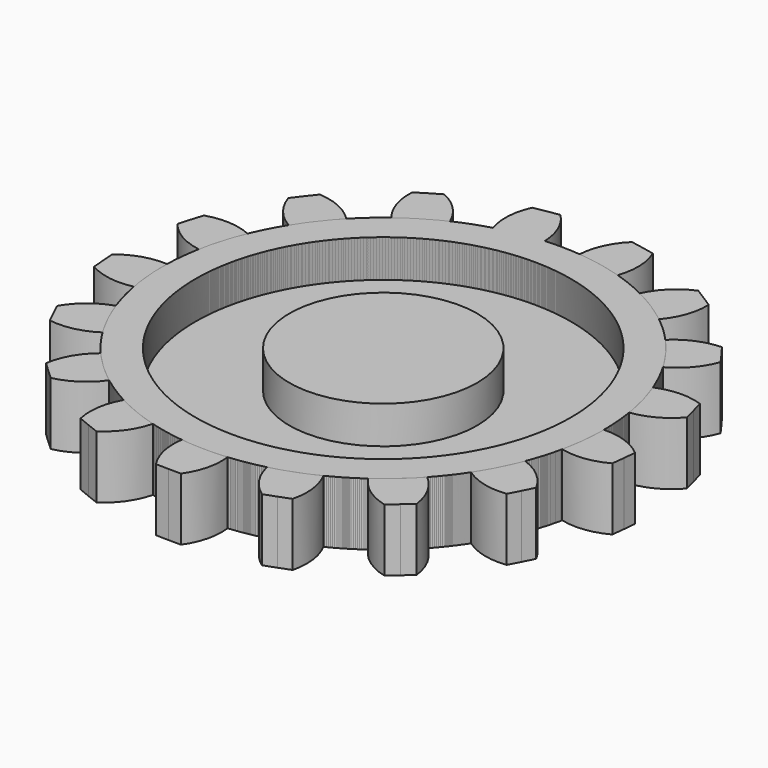
from build123d import *

# Parameters (mm, degrees)
F1_DEPTH = 5
F2_R     = 15
F2_R_2   = 7.5
F3_DEPTH = 3
F4_COUNT = 17


with BuildPart() as f1:
    # F0 (on Top) → F1 (new body)
    with BuildSketch(Plane.XY):
        with BuildLine():
            ThreePointArc((22.0684236923, 20.7148810421), (7.4013809403, -8.7073840306), (38.0585547647, 3.1639898662))
            ThreePointArc((38.0585547647, 3.1639898662), (34.6340429626, 13.6043387394), (25.691107164, 19.9880731465))
            ThreePointArc((25.691107164, 19.9880731465), (24.8010047034, 20.2408949658), (23.8988616201, 20.446659686))
            ThreePointArc((23.8988616201, 20.446659686), (22.9871638587, 20.6048003021), (22.0684236923, 20.7148810421))
        make_face()
        with BuildLine():
            ThreePointArc((23.8988616201, 20.446659686), (24.8010047034, 20.2408949658), (25.691107164, 19.9880731465))
            ThreePointArc((25.691107164, 19.9880731465), (25.9736763379, 21.8286434609), (25.570041346, 23.6465057258))
            Line((25.570041346, 23.6465057258), (24.5826281607, 23.8548088819))
            Line((24.5826281607, 23.8548088819), (23.8988616201, 20.446659686))
        make_face()
        with BuildLine():
            ThreePointArc((23.5912799835, 24.0434985608), (22.5176810984, 22.5220092068), (22.0684236923, 20.7148810421))
            ThreePointArc((22.0684236923, 20.7148810421), (22.9871638587, 20.6048003021), (23.8988616201, 20.446659686))
            Line((23.8988616201, 20.446659686), (24.5826281607, 23.8548088819))
            Line((24.5826281607, 23.8548088819), (23.5912799835, 24.0434985608))
        make_face()
    extrude(amount=F1_DEPTH)

    # F2 (on face) → F3 (cut)
    with BuildSketch(Plane.XY.offset(5)):
        with Locations((20.4314924777, 3.1639898662)):
            Circle(F2_R)
        with Locations((20.4314924777, 3.1639898662)):
            Circle(F2_R_2, mode=Mode.SUBTRACT)
    extrude(amount=-F3_DEPTH, mode=Mode.SUBTRACT)


with BuildPart() as f4_1:
    # F4: instance of F1
    add(f1.part.rotate(Axis((20.4314924777, 3.1639898662, 0), (0, 0, -1)), 1 * 360 / F4_COUNT))


with BuildPart() as f4_2:
    # F4: instance of F1
    add(f1.part.rotate(Axis((20.4314924777, 3.1639898662, 0), (0, 0, -1)), 2 * 360 / F4_COUNT))


with BuildPart() as f4_3:
    # F4: instance of F1
    add(f1.part.rotate(Axis((20.4314924777, 3.1639898662, 0), (0, 0, -1)), 3 * 360 / F4_COUNT))


with BuildPart() as f4_4:
    # F4: instance of F1
    add(f1.part.rotate(Axis((20.4314924777, 3.1639898662, 0), (0, 0, -1)), 4 * 360 / F4_COUNT))


with BuildPart() as f4_5:
    # F4: instance of F1
    add(f1.part.rotate(Axis((20.4314924777, 3.1639898662, 0), (0, 0, -1)), 5 * 360 / F4_COUNT))


with BuildPart() as f4_6:
    # F4: instance of F1
    add(f1.part.rotate(Axis((20.4314924777, 3.1639898662, 0), (0, 0, -1)), 6 * 360 / F4_COUNT))


with BuildPart() as f4_7:
    # F4: instance of F1
    add(f1.part.rotate(Axis((20.4314924777, 3.1639898662, 0), (0, 0, -1)), 7 * 360 / F4_COUNT))


with BuildPart() as f4_8:
    # F4: instance of F1
    add(f1.part.rotate(Axis((20.4314924777, 3.1639898662, 0), (0, 0, -1)), 8 * 360 / F4_COUNT))


with BuildPart() as f4_9:
    # F4: instance of F1
    add(f1.part.rotate(Axis((20.4314924777, 3.1639898662, 0), (0, 0, -1)), 9 * 360 / F4_COUNT))


with BuildPart() as f4_10:
    # F4: instance of F1
    add(f1.part.rotate(Axis((20.4314924777, 3.1639898662, 0), (0, 0, -1)), 10 * 360 / F4_COUNT))


with BuildPart() as f4_11:
    # F4: instance of F1
    add(f1.part.rotate(Axis((20.4314924777, 3.1639898662, 0), (0, 0, -1)), 11 * 360 / F4_COUNT))


with BuildPart() as f4_12:
    # F4: instance of F1
    add(f1.part.rotate(Axis((20.4314924777, 3.1639898662, 0), (0, 0, -1)), 12 * 360 / F4_COUNT))


with BuildPart() as f4_13:
    # F4: instance of F1
    add(f1.part.rotate(Axis((20.4314924777, 3.1639898662, 0), (0, 0, -1)), 13 * 360 / F4_COUNT))


with BuildPart() as f4_14:
    # F4: instance of F1
    add(f1.part.rotate(Axis((20.4314924777, 3.1639898662, 0), (0, 0, -1)), 14 * 360 / F4_COUNT))


with BuildPart() as f4_15:
    # F4: instance of F1
    add(f1.part.rotate(Axis((20.4314924777, 3.1639898662, 0), (0, 0, -1)), 15 * 360 / F4_COUNT))


with BuildPart() as f4_16:
    # F4: instance of F1
    add(f1.part.rotate(Axis((20.4314924777, 3.1639898662, 0), (0, 0, -1)), 16 * 360 / F4_COUNT))


solid = Compound([f1.part, f4_1.part, f4_2.part, f4_3.part, f4_4.part, f4_5.part, f4_6.part, f4_7.part, f4_8.part, f4_9.part, f4_10.part, f4_11.part, f4_12.part, f4_13.part, f4_14.part, f4_15.part, f4_16.part])
